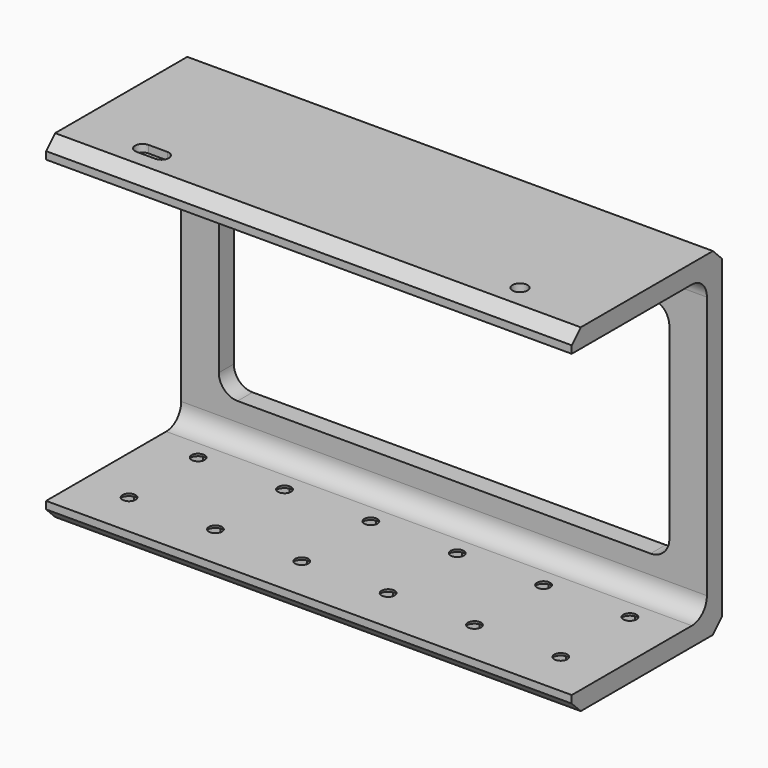
from build123d import *

# Parameters (mm, degrees)
F1_DEPTH  = 140
F3_R      = 1.75
F4_DEPTH  = 89.001
F6_DEPTH  = 4
F7_R      = 0.99999
F8_R      = 5
F9_SIZE   = 3
F11_W     = 120
F11_H     = 60
F12_DEPTH = 5.001
F13_R     = 5
F14_R     = 2
F15_DEPTH = 5
F16_R     = 3
F17_DEPTH = 3


# Not quite as in the source:
# - a fillet or chamfer is up to 0.001 mm smaller than in the source, because OpenCascade refuses the exact size


with BuildPart() as f1:
    # F0 (on Right) → F1 (new body)
    with BuildSketch(Plane.YZ):
        Polygon((-50, 5), (-50, 0), (0, 0), (0, 90), (-50, 90), (-50, 85), (-5, 85), (-5, 5), align=None)
    extrude(amount=F1_DEPTH)

    # F3 (on offset) → F4 (cut, through all)
    with BuildSketch(Plane.XY.offset(89)):
        with Locations((12.5, -38)):
            Circle(F3_R)
        with Locations((12.5, -15)):
            Circle(F3_R)
        with Locations((35.5, -38)):
            Circle(F3_R)
        with Locations((35.5, -15)):
            Circle(F3_R)
        with Locations((58.5, -38)):
            Circle(F3_R)
        with Locations((58.5, -15)):
            Circle(F3_R)
        with Locations((81.5, -38)):
            Circle(F3_R)
        with Locations((81.5, -15)):
            Circle(F3_R)
        with Locations((104.5, -38)):
            Circle(F3_R)
        with Locations((104.5, -15)):
            Circle(F3_R)
        with Locations((127.5, -38)):
            Circle(F3_R)
        with Locations((127.5, -15)):
            Circle(F3_R)
    extrude(amount=-F4_DEPTH, mode=Mode.SUBTRACT)

    # F5 (on face) → F6 (cut)
    with BuildSketch(Plane(origin=(0, 0, 0), x_dir=(1, 0, 0), z_dir=(0, 0, -1))):
        Polygon((15.9641016151, 9), (19.4282032303, 15), (15.9641016151, 21), (9.0358983849, 21), (5.5717967697, 15), (9.0358983849, 9), align=None)
        Polygon((5.5717967697, 38), (9.0358983849, 32), (15.9641016151, 32), (19.4282032303, 38), (15.9641016151, 44), (9.0358983849, 44), align=None)
        Polygon((28.5717967697, 15), (32.0358983849, 9), (38.9641016151, 9), (42.4282032303, 15), (38.9641016151, 21), (32.0358983849, 21), align=None)
        Polygon((28.5717967697, 38), (32.0358983849, 32), (38.9641016151, 32), (42.4282032303, 38), (38.9641016151, 44), (32.0358983849, 44), align=None)
        Polygon((51.5717967697, 15), (55.0358983849, 9), (61.9641016151, 9), (65.4282032303, 15), (61.9641016151, 21), (55.0358983849, 21), align=None)
        Polygon((51.5717967697, 38), (55.0358983849, 32), (61.9641016151, 32), (65.4282032303, 38), (61.9641016151, 44), (55.0358983849, 44), align=None)
        Polygon((74.5717967697, 15), (78.0358983849, 9), (84.9641016151, 9), (88.4282032303, 15), (84.9641016151, 21), (78.0358983849, 21), align=None)
        Polygon((74.5717967697, 38), (78.0358983849, 32), (84.9641016151, 32), (88.4282032303, 38), (84.9641016151, 44), (78.0358983849, 44), align=None)
        Polygon((97.5717967697, 15), (101.0358983849, 9), (107.9641016151, 9), (111.4282032303, 15), (107.9641016151, 21), (101.0358983849, 21), align=None)
        Polygon((97.5717967697, 38), (101.0358983849, 32), (107.9641016151, 32), (111.4282032303, 38), (107.9641016151, 44), (101.0358983849, 44), align=None)
        Polygon((120.5717967697, 15), (124.0358983849, 9), (130.9641016151, 9), (134.4282032303, 15), (130.9641016151, 21), (124.0358983849, 21), align=None)
        Polygon((120.5717967697, 38), (124.0358983849, 32), (130.9641016151, 32), (134.4282032303, 38), (130.9641016151, 44), (124.0358983849, 44), align=None)
    extrude(amount=-F6_DEPTH, mode=Mode.SUBTRACT)

    # F7 (radius 1 in the source; OpenCascade refuses exactly that, so slightly less here)
    f7_edges = [f1.edges().sort_by_distance(p)[0] for p in [
        (17.696152, -12, 4),
        (12.5, -9, 4),
        (17.696152, -18, 4),
        (7.303848, -12, 4),
        (12.5, -21, 4),
        (7.303848, -18, 4),
        (10.75, -15, 4),
        (7.303848, -41, 4),
        (12.5, -44, 4),
        (7.303848, -35, 4),
        (17.696152, -41, 4),
        (12.5, -32, 4),
        (17.696152, -35, 4),
        (10.75, -38, 4),
        (30.303848, -18, 4),
        (35.5, -21, 4),
        (30.303848, -12, 4),
        (40.696152, -18, 4),
        (35.5, -9, 4),
        (40.696152, -12, 4),
        (33.75, -15, 4),
        (30.303848, -41, 4),
        (35.5, -44, 4),
        (30.303848, -35, 4),
        (40.696152, -41, 4),
        (35.5, -32, 4),
        (40.696152, -35, 4),
        (33.75, -38, 4),
        (53.303848, -18, 4),
        (58.5, -21, 4),
        (53.303848, -12, 4),
        (63.696152, -18, 4),
        (58.5, -9, 4),
        (63.696152, -12, 4),
        (56.75, -15, 4),
        (53.303848, -41, 4),
        (58.5, -44, 4),
        (53.303848, -35, 4),
        (63.696152, -41, 4),
        (58.5, -32, 4),
        (63.696152, -35, 4),
        (56.75, -38, 4),
        (76.303848, -41, 4),
        (81.5, -44, 4),
        (76.303848, -35, 4),
        (86.696152, -41, 4),
        (81.5, -32, 4),
        (86.696152, -35, 4),
        (79.75, -38, 4),
        (76.303848, -18, 4),
        (81.5, -21, 4),
        (76.303848, -12, 4),
        (86.696152, -18, 4),
        (81.5, -9, 4),
        (86.696152, -12, 4),
        (79.75, -15, 4),
        (99.303848, -18, 4),
        (104.5, -21, 4),
        (99.303848, -12, 4),
        (109.696152, -18, 4),
        (104.5, -9, 4),
        (109.696152, -12, 4),
        (102.75, -15, 4),
        (99.303848, -41, 4),
        (104.5, -44, 4),
        (99.303848, -35, 4),
        (109.696152, -41, 4),
        (104.5, -32, 4),
        (109.696152, -35, 4),
        (102.75, -38, 4),
        (122.303848, -41, 4),
        (127.5, -44, 4),
        (122.303848, -35, 4),
        (132.696152, -41, 4),
        (127.5, -32, 4),
        (132.696152, -35, 4),
        (125.75, -38, 4),
        (122.303848, -18, 4),
        (127.5, -21, 4),
        (122.303848, -12, 4),
        (132.696152, -18, 4),
        (127.5, -9, 4),
        (132.696152, -12, 4),
        (125.75, -15, 4),
    ]]
    fillet(f7_edges, radius=F7_R)

    # F8
    f8_edges = [f1.edges().sort_by_distance(p)[0] for p in [
        (70, -5, 5),
        (70, -5, 85),
    ]]
    fillet(f8_edges, radius=F8_R)

    # F9
    f9_edges = [f1.edges().sort_by_distance(p)[0] for p in [
        (70, 0, 90),
        (70, -50, 90),
        (70, 0, 0),
        (70, -50, 0),
    ]]
    chamfer(f9_edges, length=F9_SIZE)

    # F11 (on face) → F12 (cut, through all)
    with BuildSketch(Plane.XZ.offset(5)):
        with Locations((70, 45)):
            Rectangle(F11_W, F11_H)
    extrude(amount=-F12_DEPTH, mode=Mode.SUBTRACT)

    # F13
    f13_edges = [f1.edges().sort_by_distance(p)[0] for p in [
        (130, -2.5, 15),
        (10, -2.5, 15),
        (130, -2.5, 75),
        (10, -2.5, 75),
    ]]
    fillet(f13_edges, radius=F13_R)

    # F14 (on face) → F15 (cut, through all)
    with BuildSketch(Plane.XY.offset(90)):
        with Locations((119, -41)):
            Circle(F14_R)
        with BuildLine():
            ThreePointArc((18.5, -39), (16.5, -41), (18.5, -43))
            Line((18.5, -43), (23.5, -43))
            ThreePointArc((23.5, -43), (25.5, -41), (23.5, -39))
            Line((23.5, -39), (18.5, -39))
        make_face()
    extrude(amount=-F15_DEPTH, mode=Mode.SUBTRACT)

    # F16 (on face) → F17 (cut)
    with BuildSketch(Plane(origin=(0, 0, 85), x_dir=(1, 0, 0), z_dir=(0, 0, -1))):
        with Locations((119, 41)):
            Circle(F16_R)
        with BuildLine():
            ThreePointArc((23.5, 38), (26.5, 41), (23.5, 44))
            Line((23.5, 44), (18.5, 44))
            ThreePointArc((18.5, 44), (15.5, 41), (18.5, 38))
            Line((18.5, 38), (23.5, 38))
        make_face()
    extrude(amount=-F17_DEPTH, mode=Mode.SUBTRACT)


solid = f1.part
